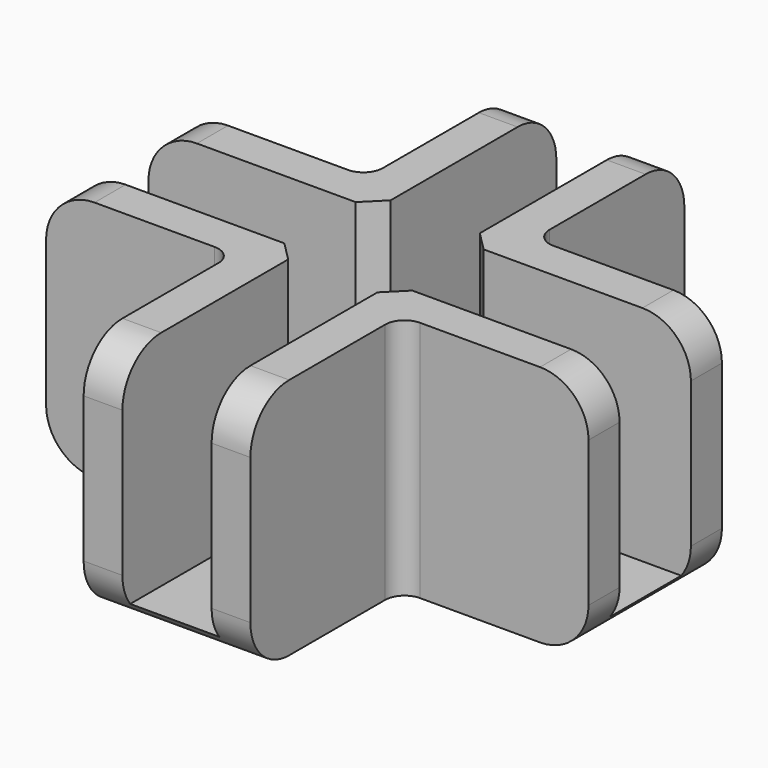
from build123d import *

# Parameters (mm, degrees)
F1_DEPTH       = 2
F2_DEPTH       = 25
F3_R           = 2
F4_T1_DEPTH    = 4
F4_T3_DEPTH    = 4
F4_T5_DEPTH    = 4
F4_T7_DEPTH    = 17.2
F4_T9_DEPTH    = 17.2
F4_T11_DEPTH   = 4
F5_R           = 2
F6_SIZE        = 2
F8_D           = 3.3
F8_CSINK_D     = 6
F8_CSINK_ANGLE = 90


# Not quite as in the source:
# - a fillet or chamfer that OpenCascade refuses, or shapes differently, is made with other operations: its cross-section is extruded or revolved along the edge and cut away or added
# - a feature names something its author has since deleted; it is built from what else it names


with BuildPart() as f1:
    # F0 (on Top) → F1 (new body)
    with BuildSketch(Plane.XY):
        Polygon((28.2951036699, 0), (28.2951036699, 9.2), (4.9215265818, 9.2), (4.9215265818, 32.5735770881), (-4.2784734182, 32.5735770881), (-4.2784734182, 9.2), (-27.6520505063, 9.2), (-27.6520505063, 0), (-4.2784734182, 0), (-4.2784734182, -23.3735770881), (4.9215265818, -23.3735770881), (4.9215265818, 0), align=None)
        Polygon((4.9215265818, 9.2), (28.2951036699, 9.2), (28.2951036699, 13.2), (8.9215265818, 13.2), (8.9215265818, 32.5735770881), (4.9215265818, 32.5735770881), align=None)
        Polygon((28.2951036699, -4), (28.2951036699, 0), (4.9215265818, 0), (4.9215265818, -23.3735770881), (8.9215265818, -23.3735770881), (8.9215265818, -4), align=None)
        Polygon((-4.2784734182, 9.2), (-4.2784734182, 32.5735770881), (-8.2784734182, 32.5735770881), (-8.2784734182, 13.2), (-27.6520505063, 13.2), (-27.6520505063, 9.2), align=None)
        Polygon((-8.2784734182, -23.3735770881), (-4.2784734182, -23.3735770881), (-4.2784734182, 0), (-27.6520505063, 0), (-27.6520505063, -4), (-8.2784734182, -4), align=None)
    extrude(amount=F1_DEPTH)

    # F0 (on Top) → F2 (join)
    with BuildSketch(Plane.XY):
        Polygon((-4.2784734182, 9.2), (-4.2784734182, 32.5735770881), (-8.2784734182, 32.5735770881), (-8.2784734182, 13.2), (-27.6520505063, 13.2), (-27.6520505063, 9.2), align=None)
        Polygon((4.9215265818, 9.2), (28.2951036699, 9.2), (28.2951036699, 13.2), (8.9215265818, 13.2), (8.9215265818, 32.5735770881), (4.9215265818, 32.5735770881), align=None)
        Polygon((-8.2784734182, -23.3735770881), (-4.2784734182, -23.3735770881), (-4.2784734182, 0), (-27.6520505063, 0), (-27.6520505063, -4), (-8.2784734182, -4), align=None)
        Polygon((28.2951036699, -4), (28.2951036699, 0), (4.9215265818, 0), (4.9215265818, -23.3735770881), (8.9215265818, -23.3735770881), (8.9215265818, -4), align=None)
    extrude(amount=F2_DEPTH)

    # F3
    f3_edges = [f1.edges().sort_by_distance(p)[0] for p in [
        (8.921527, 13.2, 12.5),
        (8.921527, -4, 12.5),
    ]]
    fillet(f3_edges, radius=F3_R)

    # F4: fillet of radius 5 on 12 edges, made by hand

    # F4_s2 → F4_t1 (cut)
    with BuildSketch(Plane.XZ.offset(-13.2)):
        with BuildLine():
            ThreePointArc((23.2951036699, 25), (26.8306375758, 23.5355339059), (28.2951036699, 20))
            Line((28.2951036699, 20), (28.3951036699, 20))
            Line((28.3951036699, 20), (28.3951036699, 25.1))
            Line((28.3951036699, 25.1), (23.2951036699, 25.1))
            Line((23.2951036699, 25.1), (23.2951036699, 25))
        make_face()
        with BuildLine():
            ThreePointArc((-27.6520505063, 20), (-26.1875844123, 23.5355339059), (-22.6520505063, 25))
            Line((-22.6520505063, 25), (-22.6520505063, 25.1))
            Line((-22.6520505063, 25.1), (-27.7520505063, 25.1))
            Line((-27.7520505063, 25.1), (-27.7520505063, 20))
            Line((-27.7520505063, 20), (-27.6520505063, 20))
        make_face()
    extrude(amount=F4_T1_DEPTH, mode=Mode.SUBTRACT)

    # F4_s4 → F4_t3 (cut)
    with BuildSketch(Plane.YZ.offset(-8.2784734182)):
        with BuildLine():
            ThreePointArc((32.5735770881, 20), (31.1091109941, 23.5355339059), (27.5735770881, 25))
            Line((27.5735770881, 25), (27.5735770881, 25.1))
            Line((27.5735770881, 25.1), (32.6735770881, 25.1))
            Line((32.6735770881, 25.1), (32.6735770881, 20))
            Line((32.6735770881, 20), (32.5735770881, 20))
        make_face()
        with BuildLine():
            ThreePointArc((-23.3735770881, 20), (-21.9091109941, 23.5355339059), (-18.3735770881, 25))
            Line((-18.3735770881, 25), (-18.3735770881, 25.1))
            Line((-18.3735770881, 25.1), (-23.4735770881, 25.1))
            Line((-23.4735770881, 25.1), (-23.4735770881, 20))
            Line((-23.4735770881, 20), (-23.3735770881, 20))
        make_face()
    extrude(amount=F4_T3_DEPTH, mode=Mode.SUBTRACT)

    # F4_s6 → F4_t5 (cut)
    with BuildSketch(Plane.YZ.offset(4.9215265818)):
        with BuildLine():
            ThreePointArc((27.5735770881, 25), (31.1091109941, 23.5355339059), (32.5735770881, 20))
            Line((32.5735770881, 20), (32.6735770881, 20))
            Line((32.6735770881, 20), (32.6735770881, 25.1))
            Line((32.6735770881, 25.1), (27.5735770881, 25.1))
            Line((27.5735770881, 25.1), (27.5735770881, 25))
        make_face()
        with BuildLine():
            ThreePointArc((-18.3735770881, 25), (-21.9091109941, 23.5355339059), (-23.3735770881, 20))
            Line((-23.3735770881, 20), (-23.4735770881, 20))
            Line((-23.4735770881, 20), (-23.4735770881, 25.1))
            Line((-23.4735770881, 25.1), (-18.3735770881, 25.1))
            Line((-18.3735770881, 25.1), (-18.3735770881, 25))
        make_face()
    extrude(amount=F4_T5_DEPTH, mode=Mode.SUBTRACT)

    # F4_s8 → F4_t7 (cut)
    with BuildSketch(Plane.XZ.offset(-13.2)):
        with BuildLine():
            ThreePointArc((-22.6520505063, 0), (-26.1875844123, 1.4644660941), (-27.6520505063, 5))
            Line((-27.6520505063, 5), (-27.7520505063, 5))
            Line((-27.7520505063, 5), (-27.7520505063, -0.1))
            Line((-27.7520505063, -0.1), (-22.6520505063, -0.1))
            Line((-22.6520505063, -0.1), (-22.6520505063, 0))
        make_face()
        with BuildLine():
            ThreePointArc((28.2951036699, 5), (26.8306375758, 1.4644660941), (23.2951036699, 0))
            Line((23.2951036699, 0), (23.2951036699, -0.1))
            Line((23.2951036699, -0.1), (28.3951036699, -0.1))
            Line((28.3951036699, -0.1), (28.3951036699, 5))
            Line((28.3951036699, 5), (28.2951036699, 5))
        make_face()
    extrude(amount=F4_T7_DEPTH, mode=Mode.SUBTRACT)

    # F4_s10 → F4_t9 (cut)
    with BuildSketch(Plane.YZ.offset(-8.2784734182)):
        with BuildLine():
            ThreePointArc((27.5735770881, 0), (31.1091109941, 1.4644660941), (32.5735770881, 5))
            Line((32.5735770881, 5), (32.6735770881, 5))
            Line((32.6735770881, 5), (32.6735770881, -0.1))
            Line((32.6735770881, -0.1), (27.5735770881, -0.1))
            Line((27.5735770881, -0.1), (27.5735770881, 0))
        make_face()
        with BuildLine():
            ThreePointArc((-18.3735770881, 0), (-21.9091109941, 1.4644660941), (-23.3735770881, 5))
            Line((-23.3735770881, 5), (-23.4735770881, 5))
            Line((-23.4735770881, 5), (-23.4735770881, -0.1))
            Line((-23.4735770881, -0.1), (-18.3735770881, -0.1))
            Line((-18.3735770881, -0.1), (-18.3735770881, 0))
        make_face()
    extrude(amount=F4_T9_DEPTH, mode=Mode.SUBTRACT)

    # F4_s12 → F4_t11 (cut)
    with BuildSketch(Plane.XZ):
        with BuildLine():
            ThreePointArc((28.2951036699, 20), (26.8306375758, 23.5355339059), (23.2951036699, 25))
            Line((23.2951036699, 25), (23.2951036699, 25.1))
            Line((23.2951036699, 25.1), (28.3951036699, 25.1))
            Line((28.3951036699, 25.1), (28.3951036699, 20))
            Line((28.3951036699, 20), (28.2951036699, 20))
        make_face()
        with BuildLine():
            ThreePointArc((-27.6520505063, 20), (-26.1875844123, 23.5355339059), (-22.6520505063, 25))
            Line((-22.6520505063, 25), (-22.6520505063, 25.1))
            Line((-22.6520505063, 25.1), (-27.7520505063, 25.1))
            Line((-27.7520505063, 25.1), (-27.7520505063, 20))
            Line((-27.7520505063, 20), (-27.6520505063, 20))
        make_face()
    extrude(amount=F4_T11_DEPTH, mode=Mode.SUBTRACT)

    # F5
    f5_edges = [f1.edges().sort_by_distance(p)[0] for p in [
        (-8.278473, 13.2, 12.5),
        (-8.278473, -4, 12.5),
    ]]
    fillet(f5_edges, radius=F5_R)

    # F6
    f6_edges = [f1.edges().sort_by_distance(p)[0] for p in [
        (4.921527, 9.2, 13.5),
        (-4.278473, 9.2, 13.5),
        (4.921527, 0, 13.5),
        (-4.278473, 0, 13.5),
    ]]
    chamfer(f6_edges, length=F6_SIZE)

    # F8 (through all)
    with Locations(Plane(origin=(0, 0, 0), x_dir=(1, 0, 0), z_dir=(0, 0, -1))):
        with Locations((0, 10.087961331), (-15, -4.6), (15, -4.6), (0, -19.6)):
            CounterSinkHole(F8_D / 2, F8_CSINK_D / 2, counter_sink_angle=F8_CSINK_ANGLE)


solid = f1.part
